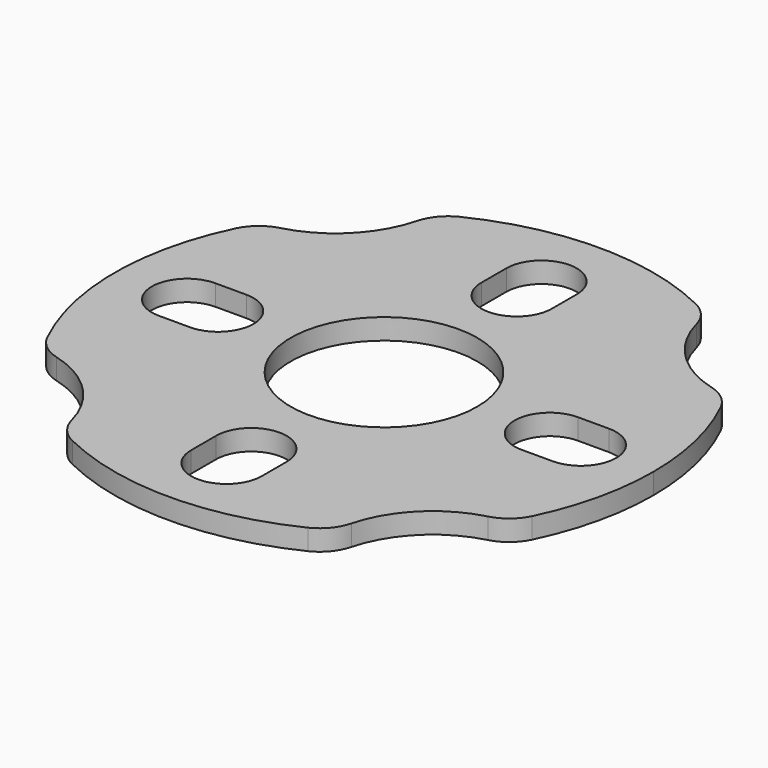
from build123d import *

# Parameters (mm, degrees)
F2_R     = 4.5
F3_DEPTH = 1
F4_R     = 2


with BuildPart() as f3:
    # F2 (on Top) → F3 (new body)
    with BuildSketch(Plane.XY):
        with BuildLine():
            ThreePointArc((11.2, -6.6), (12.5419296761, -3.4205262753), (13, 0))
            ThreePointArc((13, 0), (12.5419296761, 3.4205262753), (11.2, 6.6))
            ThreePointArc((11.2, 6.6), (8.0806476452, 8.0806476452), (6.6, 11.2))
            ThreePointArc((6.6, 11.2), (0, 13), (-6.6, 11.2))
            ThreePointArc((-6.6, 11.2), (-8.0806476452, 8.0806476452), (-11.2, 6.6))
            ThreePointArc((-11.2, 6.6), (-13, 0), (-11.2, -6.6))
            ThreePointArc((-11.2, -6.6), (-8.0806476452, -8.0806476452), (-6.6, -11.2))
            ThreePointArc((-6.6, -11.2), (0, -13), (6.6, -11.2))
            ThreePointArc((6.6, -11.2), (8.0806476452, -8.0806476452), (11.2, -6.6))
        make_face()
        with BuildLine():
            ThreePointArc((-1.7, -8), (0, -6.3), (1.7, -8))
            Line((1.7, -8), (1.7, -9.5))
            ThreePointArc((1.7, -9.5), (0, -11.2), (-1.7, -9.5))
            Line((-1.7, -9.5), (-1.7, -8))
        make_face(mode=Mode.SUBTRACT)
        with BuildLine():
            ThreePointArc((-9.5, -1.7), (-11.2, 0), (-9.5, 1.7))
            Line((-9.5, 1.7), (-8, 1.7))
            ThreePointArc((-8, 1.7), (-6.797918472, 1.202081528), (-6.3, 0))
            ThreePointArc((-6.3, 0), (-6.797918472, -1.202081528), (-8, -1.7))
            Line((-8, -1.7), (-9.5, -1.7))
        make_face(mode=Mode.SUBTRACT)
        Circle(F2_R, mode=Mode.SUBTRACT)
        with BuildLine():
            ThreePointArc((8, -1.7), (6.3, 0), (8, 1.7))
            Line((8, 1.7), (9.5, 1.7))
            ThreePointArc((9.5, 1.7), (10.702081528, 1.202081528), (11.2, 0))
            ThreePointArc((11.2, 0), (10.702081528, -1.202081528), (9.5, -1.7))
            Line((9.5, -1.7), (8, -1.7))
        make_face(mode=Mode.SUBTRACT)
        with BuildLine():
            ThreePointArc((-1.7, 9.5), (0, 11.2), (1.7, 9.5))
            Line((1.7, 9.5), (1.7, 8))
            ThreePointArc((1.7, 8), (0, 6.3), (-1.7, 8))
            Line((-1.7, 8), (-1.7, 9.5))
        make_face(mode=Mode.SUBTRACT)
    extrude(amount=F3_DEPTH)

    # F4
    f4_edges = [f3.edges().sort_by_distance(p)[0] for p in [
        (-11.2, -6.6, 0.5),
        (11.2, -6.6, 0.5),
        (11.2, 6.6, 0.5),
        (-11.2, 6.6, 0.5),
        (6.6, -11.2, 0.5),
        (-6.6, -11.2, 0.5),
        (-6.6, 11.2, 0.5),
        (6.6, 11.2, 0.5),
    ]]
    fillet(f4_edges, radius=F4_R)


solid = f3.part
